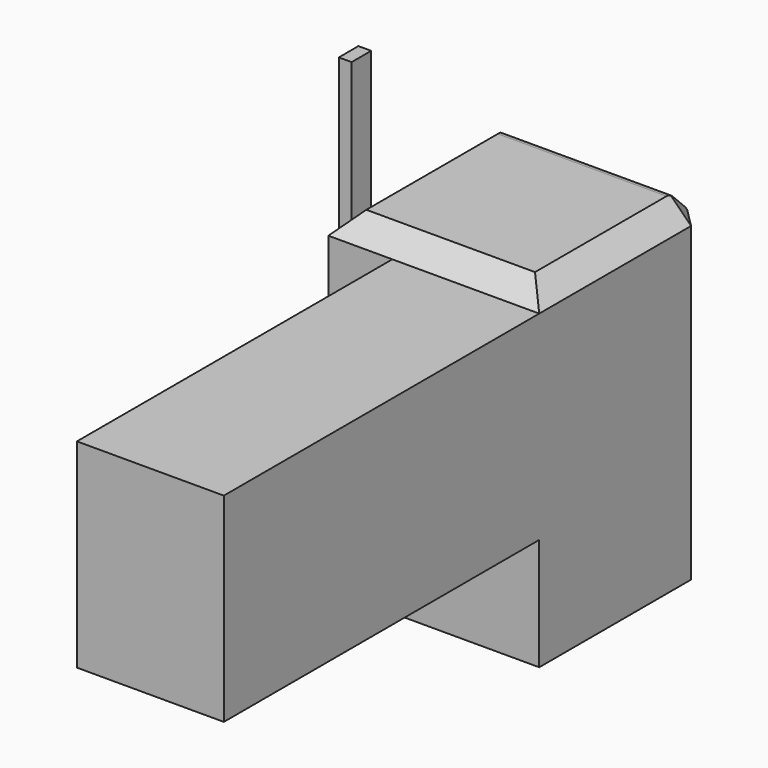
from build123d import *

# Parameters (mm, degrees)
F0_W     = 3.0842895067
F0_H     = 5.8946473162
F1_DEPTH = 80.0870582461
F0_W_2   = 50.8
F0_H_2   = 50.8
F2_SIZE  = 5.08
F3_R     = 2.54
F6_W     = 35.3883287489
F6_H     = 47.9876469207
F7_DEPTH = 94.9677098542


# Not quite as in the source:
# - the program builds the solid bodies; features that only make, move or delete a surface that nothing else refers to are left out


with BuildPart() as f1:
    # F0 (on Top) → F1 (new body)
    with BuildSketch(Plane.XY):
        with Locations((-36.1949966816, 26.8958949286)):
            Rectangle(F0_W, F0_H)
    extrude(amount=F1_DEPTH)


with BuildPart() as f1b:
    # F0 (on Top) → F1, piece 2 (new body)
    with BuildSketch(Plane.XY):
        with Locations((25.4, -0.9800925486)):
            Rectangle(F0_W_2, F0_H_2)
    extrude(amount=F1_DEPTH)

    # F2
    f2_edges = [f1b.edges().sort_by_distance(p)[0] for p in [
        (25.4, -26.380093, 80.087058),
        (0, -0.980093, 80.087058),
        (25.4, 24.419907, 80.087058),
        (50.8, -0.980093, 80.087058),
        (0, 24.419907, 40.043529),
        (25.4, 24.419907, 0),
        (50.8, 24.419907, 40.043529),
    ]]
    chamfer(f2_edges, length=F2_SIZE)

    # F3
    f3_edges = [f1b.edges().sort_by_distance(p)[0] for p in [
        (25.4, 19.339907, 80.087058),
        (25.4, 24.419907, 75.007058),
    ]]
    fillet(f3_edges, radius=F3_R)

    # F6 (on face) → F7 (join)
    with BuildSketch(Plane.XZ.offset(26.3800925486)):
        with Locations((33.1058356255, 51.0132347858)):
            Rectangle(F6_W, F6_H)
    extrude(amount=F7_DEPTH)


solid = Compound([f1.part, f1b.part])
